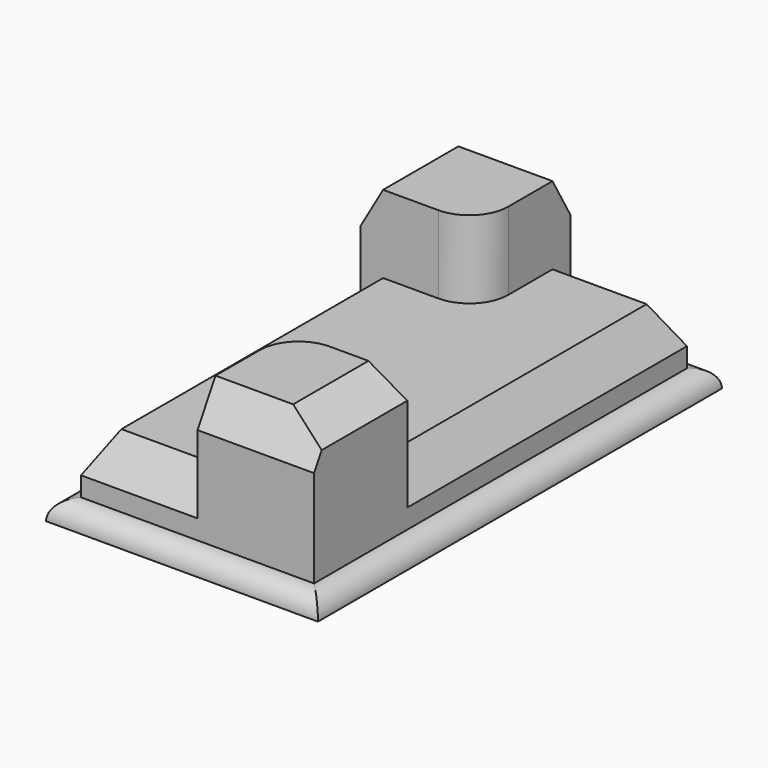
from build123d import *

# Parameters (mm, degrees)
F0_W        = 88.9
F0_H        = 165.1
F1_DEPTH    = 6.35
F2_R        = 6.34999
F3_DEPTH    = 25.4
F4_DEPTH    = 50.8
F5_C1_SIZE2 = 7.3323484187
F5_C1_SIZE  = 12.7
F5_C2_SIZE2 = 12.7
F5_C2_SIZE  = 7.3323484187
F5_C3_SIZE2 = 7.3323484187
F5_C3_SIZE  = 12.7
F5_C4_SIZE2 = 7.3323484187
F5_C4_SIZE  = 12.7
F6_C1_SIZE2 = 7.3323484187
F6_C1_SIZE  = 12.7
F6_C2_SIZE2 = 12.7
F6_C2_SIZE  = 7.3323484187
F6_C3_SIZE2 = 12.7
F6_C3_SIZE  = 7.3323484187
F6_C4_SIZE2 = 12.7
F6_C4_SIZE  = 7.3323484187


# Not quite as in the source:
# - a fillet or chamfer is up to 0.001 mm smaller than in the source, because OpenCascade refuses the exact size


with BuildPart() as f1:
    # F0 (on Top) → F1 (new body)
    with BuildSketch(Plane.XY):
        Rectangle(F0_W, F0_H)
        Polygon((-38.1, 38.1), (-38.1, 76.2), (0, 76.2), (38.1, 76.2), (38.1, -38.1), (38.1, -76.2), (0, -76.2), (-38.1, -76.2), align=None, mode=Mode.SUBTRACT)
    extrude(amount=F1_DEPTH)

    # F2 (radius 6.35 in the source; OpenCascade refuses exactly that, so slightly less here)
    f2_edges = [f1.edges().sort_by_distance(p)[0] for p in [
        (-44.45, 0, 6.35),
        (0, -82.55, 6.35),
        (44.45, 0, 6.35),
        (0, 82.55, 6.35),
    ]]
    fillet(f2_edges, radius=F2_R)

    # F0 (on Top) → F3 (join)
    with BuildSketch(Plane.XY):
        with BuildLine():
            Line((38.1, 76.2), (0, 76.2))
            Line((0, 76.2), (0, 50.8))
            ThreePointArc((0, 50.8), (-3.7197438789, 41.8197438789), (-12.7, 38.1))
            Line((-12.7, 38.1), (-38.1, 38.1))
            Line((-38.1, 38.1), (-38.1, -76.2))
            Line((-38.1, -76.2), (0, -76.2))
            Line((0, -76.2), (0, -50.8))
            ThreePointArc((0, -50.8), (3.7197438789, -41.8197438789), (12.7, -38.1))
            Line((12.7, -38.1), (38.1, -38.1))
            Line((38.1, -38.1), (38.1, 76.2))
        make_face()
    extrude(amount=F3_DEPTH)

    # F0 (on Top) → F4 (join)
    with BuildSketch(Plane.XY):
        with BuildLine():
            Line((38.1, -76.2), (38.1, -38.1))
            Line((38.1, -38.1), (12.7, -38.1))
            ThreePointArc((12.7, -38.1), (3.7197438789, -41.8197438789), (0, -50.8))
            Line((0, -50.8), (0, -76.2))
            Line((0, -76.2), (38.1, -76.2))
        make_face()
        with BuildLine():
            Line((0, 76.2), (-38.1, 76.2))
            Line((-38.1, 76.2), (-38.1, 38.1))
            Line((-38.1, 38.1), (-12.7, 38.1))
            ThreePointArc((-12.7, 38.1), (-3.7197438789, 41.8197438789), (0, 50.8))
            Line((0, 50.8), (0, 76.2))
        make_face()
    extrude(amount=F4_DEPTH)

    # F5: chamfer of 12.7 x 7.3323484187 on 4 edges, made by hand

    # F5_c1
    f5_c1_edges = [f1.edges().sort_by_distance(p)[0] for p in [
        (19.05, -76.2, 50.8),
    ]]
    f5_c1_side = f1.faces().sort_by_distance((19.05, -76.2, 50.6533530316))[0]
    chamfer(f5_c1_edges, length=F5_C1_SIZE, length2=F5_C1_SIZE2, reference=f5_c1_side)

    # F5_c2
    f5_c2_edges = [f1.edges().sort_by_distance(p)[0] for p in [
        (38.1, -53.4838257906, 50.8),
    ]]
    f5_c2_side = f1.faces().sort_by_distance((38.1, -53.4838257906, 50.6533530316))[0]
    chamfer(f5_c2_edges, length=F5_C2_SIZE, length2=F5_C2_SIZE2, reference=f5_c2_side)

    # F5_c3
    f5_c3_edges = [f1.edges().sort_by_distance(p)[0] for p in [
        (-19.05, 76.2, 50.8),
    ]]
    f5_c3_side = f1.faces().sort_by_distance((-19.05, 76.2, 50.6533530316))[0]
    chamfer(f5_c3_edges, length=F5_C3_SIZE, length2=F5_C3_SIZE2, reference=f5_c3_side)

    # F5_c4
    f5_c4_edges = [f1.edges().sort_by_distance(p)[0] for p in [
        (-38.1, 53.4838257906, 50.8),
    ]]
    f5_c4_side = f1.faces().sort_by_distance((-38.1, 53.4838257906, 50.6533530316))[0]
    chamfer(f5_c4_edges, length=F5_C4_SIZE, length2=F5_C4_SIZE2, reference=f5_c4_side)

    # F6: chamfer of 12.7 x 7.3323484187 on 4 edges, made by hand

    # F6_c1
    f6_c1_edges = [f1.edges().sort_by_distance(p)[0] for p in [
        (19.05, 76.2, 25.4),
    ]]
    f6_c1_side = f1.faces().sort_by_distance((19.05, 76.2, 25.2533530316))[0]
    chamfer(f6_c1_edges, length=F6_C1_SIZE, length2=F6_C1_SIZE2, reference=f6_c1_side)

    # F6_c2
    f6_c2_edges = [f1.edges().sort_by_distance(p)[0] for p in [
        (-38.1, -19.05, 25.4),
    ]]
    f6_c2_side = f1.faces().sort_by_distance((-37.9533530316, -19.05, 25.4))[0]
    chamfer(f6_c2_edges, length=F6_C2_SIZE, length2=F6_C2_SIZE2, reference=f6_c2_side)

    # F6_c3
    f6_c3_edges = [f1.edges().sort_by_distance(p)[0] for p in [
        (38.1, 15.3838257906, 25.4),
    ]]
    f6_c3_side = f1.faces().sort_by_distance((37.9533530316, 15.3838257906, 25.4))[0]
    chamfer(f6_c3_edges, length=F6_C3_SIZE, length2=F6_C3_SIZE2, reference=f6_c3_side)

    # F6_c4
    f6_c4_edges = [f1.edges().sort_by_distance(p)[0] for p in [
        (-15.3838257906, -76.2, 25.4),
    ]]
    f6_c4_side = f1.faces().sort_by_distance((-15.3838257906, -76.0533530316, 25.4))[0]
    chamfer(f6_c4_edges, length=F6_C4_SIZE, length2=F6_C4_SIZE2, reference=f6_c4_side)


solid = f1.part
